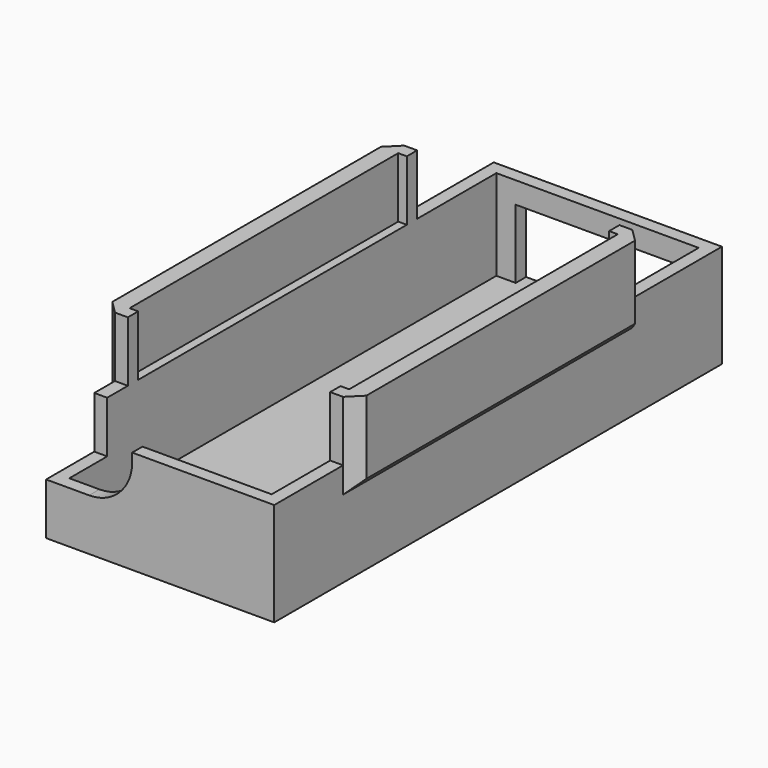
from build123d import *

# Parameters (mm, degrees)
F0_W      = 23.5
F0_H      = 62
F1_DEPTH  = 1.5
F2_W      = 26.5
F2_H      = 65
F2_W_2    = 23.5
F2_H_2    = 62
F3_DEPTH  = 12
F4_W      = 2
F4_H      = 39
F5_DEPTH  = 7
F7_DEPTH  = 7
F8_W      = 19
F8_H      = 5
F9_DEPTH  = 8
F11_DEPTH = 6
F12_R     = 5
F13_DEPTH = 3
F14_SIZE  = 1.49999


# Not quite as in the source:
# - a fillet or chamfer is up to 0.001 mm smaller than in the source, because OpenCascade refuses the exact size


with BuildPart() as f1:
    # F0 (on Top) → F1 (new body)
    with BuildSketch(Plane.XY):
        Rectangle(F0_W, F0_H)
    extrude(amount=F1_DEPTH)

    # F2 (on Top) → F3 (join)
    with BuildSketch(Plane.XY):
        Rectangle(F2_W, F2_H)
        Rectangle(F2_W_2, F2_H_2, mode=Mode.SUBTRACT)
    extrude(amount=F3_DEPTH)

    # F4 (on face) → F5 (join)
    with BuildSketch(Plane.XY.offset(12)):
        with Locations((-13.75, -1.5)):
            Rectangle(F4_W, F4_H)
        with Locations((13.75, -1.5)):
            Rectangle(F4_W, F4_H)
    extrude(amount=F5_DEPTH)

    # F6 (on face) → F7 (join, through all)
    with BuildSketch(Plane.XY.offset(12)):
        Polygon((14.75, -21), (11.75, -21), (11.75, -22.5), (13.25, -22.5), align=None)
        Polygon((11.75, 19.5), (11.75, 18), (14.75, 18), (13.25, 19.5), align=None)
        Polygon((-13.25, 19.5), (-14.75, 18), (-11.75, 18), (-11.75, 19.5), align=None)
        Polygon((-11.75, -22.5), (-11.75, -21), (-14.75, -21), (-13.25, -22.5), align=None)
    extrude(amount=F7_DEPTH)

    # F8 (on face) → F9 (cut)
    with BuildSketch(Plane.XY.offset(1.5)):
        with Locations((0, 31)):
            Rectangle(F8_W, F8_H)
    extrude(amount=F9_DEPTH, mode=Mode.SUBTRACT)

    # F10 (on face) → F11 (cut)
    with BuildSketch(Plane.XY.offset(12)):
        Polygon((-13.25, -25.5), (-13.25, -32.5), (-3.25, -32.5), (-3.25, -31), (-11.75, -31), (-11.75, -25.5), align=None)
    extrude(amount=-F11_DEPTH, mode=Mode.SUBTRACT)

    # F12
    f12_edges = [f1.edges().sort_by_distance(p)[0] for p in [
        (-3.25, -31.75, 6),
    ]]
    fillet(f12_edges, radius=F12_R)

    # F13 (add): faces of the model
    f13_faces = [f1.faces().sort_by_distance(p)[0] for p in [
        (-13.9907407407, -1.5, 12),
        (13.9907407407, -1.5, 12),
    ]]
    extrude(f13_faces, amount=F13_DEPTH)

    # F14 (size 1.5 in the source; OpenCascade refuses exactly that, so slightly less here)
    f14_edges = [f1.edges().sort_by_distance(p)[0] for p in [
        (-14.75, -1.5, 9),
        (14.75, -1.5, 9),
    ]]
    chamfer(f14_edges, length=F14_SIZE)


solid = f1.part
